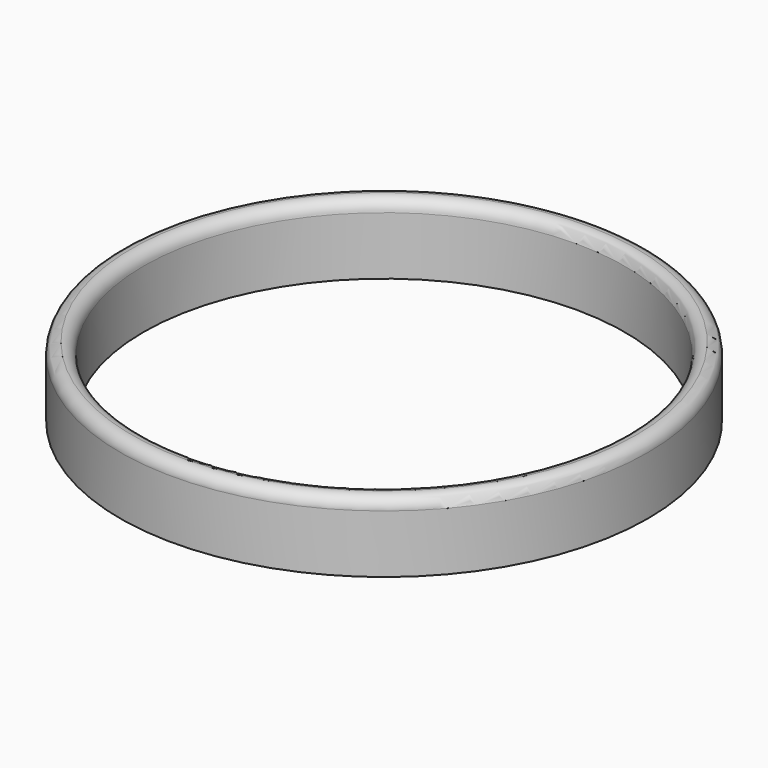
from build123d import *

# Parameters (mm, degrees)
F0_R     = 11.35
F0_R_2   = 10.35
F1_DEPTH = 3
F2_R     = 0.49999


# Not quite as in the source:
# - a fillet or chamfer is up to 0.001 mm smaller than in the source, because OpenCascade refuses the exact size


with BuildPart() as f1:
    # F0 (on Top) → F1 (new body)
    with BuildSketch(Plane.XY):
        Circle(F0_R)
        Circle(F0_R_2, mode=Mode.SUBTRACT)
    extrude(amount=F1_DEPTH)

    # F2 (radius 0.5 in the source; OpenCascade refuses exactly that, so slightly less here)
    f2_edges = [f1.edges().sort_by_distance(p)[0] for p in [
        (-11.35, 0, 3),
        (-10.35, 0, 3),
    ]]
    fillet(f2_edges, radius=F2_R)


solid = f1.part
